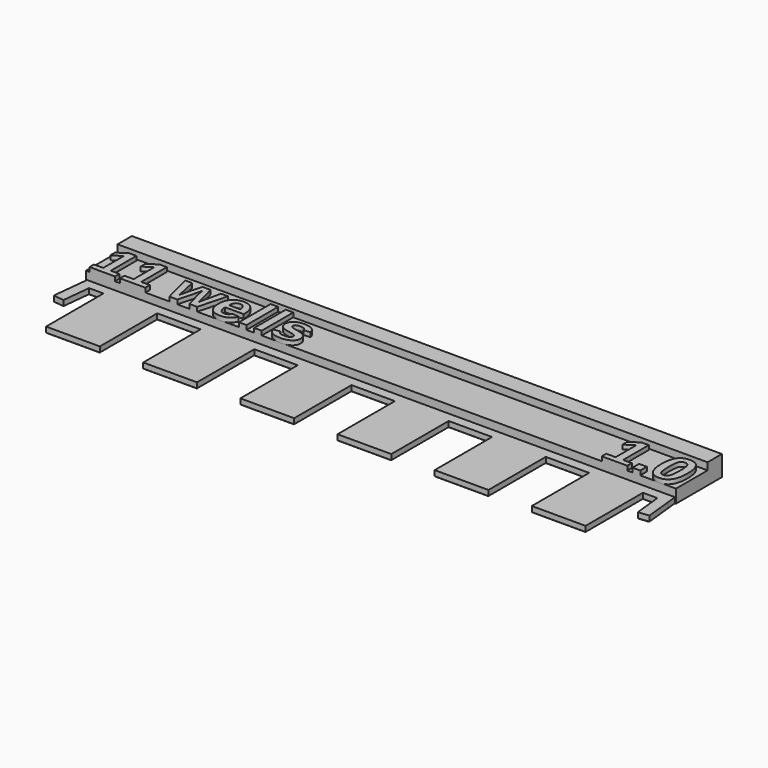
from build123d import *

# Parameters (mm, degrees)
F2_DEPTH      = 0.9
F3_DEPTH      = 2
F1_W          = 82.3
F1_H          = 2.5
F4_DEPTH      = 3
F5_TEXT_SIZE  = 7.6388888889
F6_DEPTH      = 0.6
F7_T1_DEPTH   = 2.532279032
F7_T3_DEPTH   = 10.516139516
F7_T5_DEPTH   = 8.532279032
F7_T7_DEPTH   = 6.05
F7_T9_DEPTH   = 8.532279032
F7_T11_DEPTH  = 6.05
F7_T13_DEPTH  = 8.532279032
F7_T15_DEPTH  = 6.05
F7_T17_DEPTH  = 8.532279032
F7_T19_DEPTH  = 6.05
F7_T21_DEPTH  = 8.532279032
F7_T23_DEPTH  = 6.05
F7_T25_DEPTH  = 8.532279032
F7_T27_DEPTH  = 2.532279032
F7_T29_DEPTH  = 9.032279032
F7_T31_DEPTH  = 83.332279032
F7_T36_DEPTH  = 1.1794249614
F7_T41_DEPTH  = 6.1899906234
F7_T46_DEPTH  = 4.9746099208
F7_T51_DEPTH  = 2.5292526207
F7_T56_DEPTH  = 2.5292526207
F7_T61_DEPTH  = 4.9746099208
F7_T66_DEPTH  = 6.1899906234
F7_T71_DEPTH  = 1.1794249614
F7_T77_DEPTH  = 1.1794249614
F7_T81_DEPTH  = 6.1899906234
F7_T88_DEPTH  = 4.9746099208
F7_T92_DEPTH  = 2.5292526207
F7_T99_DEPTH  = 3.0453921368
F7_T103_DEPTH = 11.032279032
F7_T110_DEPTH = 11.032279032
F7_T114_DEPTH = 6.566139516
F7_T121_DEPTH = 6.566139516
F7_T125_DEPTH = 11.032279032
F7_T132_DEPTH = 11.032279032
F7_T136_DEPTH = 6.566139516
F7_T143_DEPTH = 6.566139516
F7_T147_DEPTH = 11.032279032
F7_T154_DEPTH = 11.032279032
F7_T158_DEPTH = 6.566139516
F7_T165_DEPTH = 6.566139516
F7_T169_DEPTH = 11.032279032
F7_T176_DEPTH = 11.032279032
F7_T180_DEPTH = 6.566139516
F7_T187_DEPTH = 6.566139516
F7_T191_DEPTH = 11.032279032
F7_T198_DEPTH = 11.032279032
F7_T202_DEPTH = 6.566139516
F7_T209_DEPTH = 6.566139516
F7_T213_DEPTH = 11.032279032
F7_T220_DEPTH = 11.032279032
F7_T224_DEPTH = 3.0453921368
F7_T231_DEPTH = 2.5292526207
F7_T235_DEPTH = 4.9746099208
F7_T242_DEPTH = 1.1794249614
F7_T246_DEPTH = 6.1899906234


# Not quite as in the source:
# - a fillet or chamfer that OpenCascade refuses, or shapes differently, is made with other operations: its cross-section is extruded or revolved along the edge and cut away or added
# - Text() gives the source's letters only with a copy of the font that has no kerning and outlines rounded to 1/6400 em; it was checked with that copy


with BuildPart() as f2:
    # F1 (on Top) → F2 (new body)
    with BuildSketch(Plane.XY):
        Polygon((-34.0542682267, 5.1274530911), (-32.041155122, 5.1274530911), (-32.041155122, -4.8725469089), (-24.541155122, -4.8725469089), (-24.541155122, 5.1274530911), (-18.491155122, 5.1274530911), (-18.491155122, -4.8725469089), (-10.991155122, -4.8725469089), (-10.991155122, 5.1274530911), (-4.941155122, 5.1274530911), (-4.941155122, -4.8725469089), (2.558844878, -4.8725469089), (2.558844878, 5.1274530911), (8.608844878, 5.1274530911), (8.608844878, -4.8725469089), (16.108844878, -4.8725469089), (16.108844878, 5.1274530911), (22.158844878, 5.1274530911), (22.158844878, -4.8725469089), (29.658844878, -4.8725469089), (29.658844878, 5.1274530911), (35.708844878, 5.1274530911), (35.708844878, -4.8725469089), (43.208844878, -4.8725469089), (43.208844878, 5.1274530911), (45.2219579827, 5.1274530911), (45.6340437722, 1.2067187034), (47.1258266152, 1.3635113983), (46.733844878, 5.092968506), (46.5866989486, 6.492968506), (-35.4190091927, 6.492968506), (-35.566155122, 5.092968506), (-35.9581368593, 1.3635113983), (-34.4663540162, 1.2067187034), align=None)
    extrude(amount=F2_DEPTH)

    # F1 (on Top) → F3 (join)
    with BuildSketch(Plane.XY):
        Polygon((-35.566155122, 6.492968506), (-35.4190091927, 6.492968506), (46.5866989486, 6.492968506), (46.733844878, 6.492968506), (46.733844878, 11.992968506), (-35.566155122, 11.992968506), align=None)
    extrude(amount=F3_DEPTH)

    # F1 (on Top) → F4 (join)
    with BuildSketch(Plane.XY):
        with Locations((5.583844878, 13.242968506)):
            Rectangle(F1_W, F1_H)
    extrude(amount=F4_DEPTH)

    # F5 (on face) → F6 (join)
    with BuildSketch(Plane.XY.offset(2)):
        with Locations((35.8985584196, 6.492968506)):
            Text('1.0', F5_TEXT_SIZE, font='Arimo', font_style=FontStyle.BOLD, text_align=(TextAlign.LEFT, TextAlign.BOTTOM))
        with Locations((-35.566155122, 6.492968506)):
            Text('11 wells', F5_TEXT_SIZE, font='Arimo', font_style=FontStyle.BOLD, text_align=(TextAlign.LEFT, TextAlign.BOTTOM))
    extrude(amount=F6_DEPTH)

    # F7: chamfer of 0.15 x 0.2 on 36 edges, made by hand

    # F7_s2 → F7_t1 (cut)
    with BuildSketch(Plane(origin=(-36.2203081074, 3.8069077847, 0), x_dir=(0, 0, 1), z_dir=(0.9945218954, -0.1045284633, 0))):
        Polygon((0, 2.2026068477), (0.15, 2.4026068477), (0, 2.4026068477), align=None)
    extrude(amount=F7_T1_DEPTH, mode=Mode.SUBTRACT)

    # F7_s4 → F7_t3 (cut)
    with BuildSketch(Plane.XZ.offset(-5.1274530911)):
        Polygon((-31.841155122, 0), (-32.041155122, 0.15), (-32.041155122, 0), align=None)
        Polygon((-24.741155122, 0), (-24.541155122, 0.15), (-24.541155122, 0), align=None)
        Polygon((-18.291155122, 0), (-18.491155122, 0.15), (-18.491155122, 0), align=None)
        Polygon((-11.191155122, 0), (-10.991155122, 0.15), (-10.991155122, 0), align=None)
        Polygon((-4.741155122, 0), (-4.941155122, 0.15), (-4.941155122, 0), align=None)
        Polygon((2.358844878, 0), (2.558844878, 0.15), (2.558844878, 0), align=None)
        Polygon((8.808844878, 0), (8.608844878, 0.15), (8.608844878, 0), align=None)
        Polygon((15.908844878, 0), (16.108844878, 0.15), (16.108844878, 0), align=None)
        Polygon((22.358844878, 0), (22.158844878, 0.15), (22.158844878, 0), align=None)
        Polygon((29.458844878, 0), (29.658844878, 0.15), (29.658844878, 0), align=None)
        Polygon((35.908844878, 0), (35.708844878, 0.15), (35.708844878, 0), align=None)
        Polygon((43.008844878, 0), (43.208844878, 0.15), (43.208844878, 0), align=None)
    extrude(amount=F7_T3_DEPTH, mode=Mode.SUBTRACT)

    # F7_s6 → F7_t5 (cut)
    with BuildSketch(Plane.YZ.offset(-32.5572946381)):
        Polygon((-4.6725469089, 0), (-4.8725469089, 0.15), (-4.8725469089, 0), align=None)
    extrude(amount=F7_T5_DEPTH, mode=Mode.SUBTRACT)

    # F7_s8 → F7_t7 (cut)
    with BuildSketch(Plane.YZ.offset(-24.541155122)):
        Polygon((5.3274530911, 0), (5.1274530911, 0.15), (5.1274530911, 0), align=None)
    extrude(amount=F7_T7_DEPTH, mode=Mode.SUBTRACT)

    # F7_s10 → F7_t9 (cut)
    with BuildSketch(Plane.YZ.offset(-19.0072946381)):
        Polygon((-4.6725469089, 0), (-4.8725469089, 0.15), (-4.8725469089, 0), align=None)
    extrude(amount=F7_T9_DEPTH, mode=Mode.SUBTRACT)

    # F7_s12 → F7_t11 (cut)
    with BuildSketch(Plane.YZ.offset(-10.991155122)):
        Polygon((5.3274530911, 0), (5.1274530911, 0.15), (5.1274530911, 0), align=None)
    extrude(amount=F7_T11_DEPTH, mode=Mode.SUBTRACT)

    # F7_s14 → F7_t13 (cut)
    with BuildSketch(Plane.YZ.offset(-5.4572946381)):
        Polygon((-4.6725469089, 0), (-4.8725469089, 0.15), (-4.8725469089, 0), align=None)
    extrude(amount=F7_T13_DEPTH, mode=Mode.SUBTRACT)

    # F7_s16 → F7_t15 (cut)
    with BuildSketch(Plane.YZ.offset(2.558844878)):
        Polygon((5.3274530911, 0), (5.1274530911, 0.15), (5.1274530911, 0), align=None)
    extrude(amount=F7_T15_DEPTH, mode=Mode.SUBTRACT)

    # F7_s18 → F7_t17 (cut)
    with BuildSketch(Plane.YZ.offset(8.0927053619)):
        Polygon((-4.6725469089, 0), (-4.8725469089, 0.15), (-4.8725469089, 0), align=None)
    extrude(amount=F7_T17_DEPTH, mode=Mode.SUBTRACT)

    # F7_s20 → F7_t19 (cut)
    with BuildSketch(Plane.YZ.offset(16.108844878)):
        Polygon((5.3274530911, 0), (5.1274530911, 0.15), (5.1274530911, 0), align=None)
    extrude(amount=F7_T19_DEPTH, mode=Mode.SUBTRACT)

    # F7_s22 → F7_t21 (cut)
    with BuildSketch(Plane.YZ.offset(21.6427053619)):
        Polygon((-4.6725469089, 0), (-4.8725469089, 0.15), (-4.8725469089, 0), align=None)
    extrude(amount=F7_T21_DEPTH, mode=Mode.SUBTRACT)

    # F7_s24 → F7_t23 (cut)
    with BuildSketch(Plane.YZ.offset(29.658844878)):
        Polygon((5.3274530911, 0), (5.1274530911, 0.15), (5.1274530911, 0), align=None)
    extrude(amount=F7_T23_DEPTH, mode=Mode.SUBTRACT)

    # F7_s26 → F7_t25 (cut)
    with BuildSketch(Plane.YZ.offset(35.1927053619)):
        Polygon((-4.6725469089, 0), (-4.8725469089, 0.15), (-4.8725469089, 0), align=None)
    extrude(amount=F7_T25_DEPTH, mode=Mode.SUBTRACT)

    # F7_s28 → F7_t27 (cut)
    with BuildSketch(Plane(origin=(44.7475705131, 4.7031591788, 0), x_dir=(0, 0, 1), z_dir=(0.9945218954, 0.1045284633, 0))):
        Polygon((0, 3.3699482961), (0.15, 3.5699482961), (0, 3.5699482961), align=None)
    extrude(amount=F7_T27_DEPTH, mode=Mode.SUBTRACT)

    # F7_s30 → F7_t29 (cut)
    with BuildSketch(Plane.XZ.offset(-15.009108022)):
        Polygon((46.533844878, 0), (46.733844878, 0.15), (46.733844878, 0), align=None)
        Polygon((-35.366155122, 0), (-35.566155122, 0.15), (-35.566155122, 0), align=None)
    extrude(amount=F7_T29_DEPTH, mode=Mode.SUBTRACT)

    # F7_s32 → F7_t31 (cut)
    with BuildSketch(Plane.YZ.offset(-36.0822946381)):
        Polygon((14.292968506, 0), (14.492968506, 0.15), (14.492968506, 0), align=None)
    extrude(amount=F7_T31_DEPTH, mode=Mode.SUBTRACT)


with BuildPart() as f7_tool34:
    # F7_s35 → F7_t36 (new body)
    with BuildSketch(Plane.YZ.offset(-36.0822946381)):
        Polygon((6.492968506, 0.15), (6.692968506, 0), (6.492968506, 0), align=None)
    extrude(amount=F7_T36_DEPTH)

    split(bisect_by=Plane(origin=(-35.7069960577, 3.7529565143, 0), x_dir=(0, 0, 1), z_dir=(-0.9945218954, 0.1045284633, 0)), keep=Keep.TOP)


with BuildPart() as f2_1:
    add(f2.part)

    # F7_t33: cut F7_tool34
    add(f7_tool34.part, mode=Mode.SUBTRACT)


with BuildPart() as f7_tool39:
    # F7_s40 → F7_t41 (new body)
    with BuildSketch(Plane(origin=(0.3419381354, 3.2533240414, 0), x_dir=(0, 0, 1), z_dir=(-0.1045284633, -0.9945218954, 0))):
        Polygon((0, 35.7036801743), (0.15, 35.9036801743), (0, 35.9036801743), align=None)
    extrude(amount=F7_T41_DEPTH)

    split(bisect_by=Plane.XZ.offset(-6.492968506), keep=Keep.TOP)


with BuildPart() as f2_2:
    add(f2_1.part)

    # F7_t38: cut F7_tool39
    add(f7_tool39.part, mode=Mode.SUBTRACT)


with BuildPart() as f7_tool44:
    # F7_s45 → F7_t46 (new body)
    with BuildSketch(Plane(origin=(-0.3050920721, -2.9027571657, 0), x_dir=(0, 0, 1), z_dir=(0.1045284633, 0.9945218954, 0))):
        Polygon((0, -34.6036801743), (0.15, -34.4036801743), (0, -34.4036801743), align=None)
    extrude(amount=F7_T46_DEPTH)

    split(bisect_by=Plane.XZ.offset(-5.1274530911), keep=Keep.TOP)


with BuildPart() as f2_3:
    add(f2_2.part)

    # F7_t43: cut F7_tool44
    add(f7_tool44.part, mode=Mode.SUBTRACT)


with BuildPart() as f7_tool49:
    # F7_s50 → F7_t51 (new body)
    with BuildSketch(Plane.YZ.offset(-34.5704077428)):
        Polygon((5.3274530911, 0), (5.1274530911, 0.15), (5.1274530911, 0), align=None)
    extrude(amount=F7_T51_DEPTH)

    split(bisect_by=Plane(origin=(-34.2152132146, 3.5961638194, 0), x_dir=(0, 0, 1), z_dir=(0.9945218954, -0.1045284633, 0)), keep=Keep.TOP)


with BuildPart() as f2_4:
    add(f2_3.part)

    # F7_t48: cut F7_tool49
    add(f7_tool49.part, mode=Mode.SUBTRACT)


with BuildPart() as f7_tool54:
    # F7_s55 → F7_t56 (new body)
    with BuildSketch(Plane.YZ.offset(43.208844878)):
        Polygon((5.3274530911, 0), (5.1274530911, 0.15), (5.1274530911, 0), align=None)
    extrude(amount=F7_T56_DEPTH)

    split(bisect_by=Plane(origin=(45.2608825628, 4.7571104492, 0), x_dir=(0, 0, 1), z_dir=(-0.9945218954, -0.1045284633, 0)), keep=Keep.TOP)


with BuildPart() as f2_5:
    add(f2_4.part)

    # F7_t53: cut F7_tool54
    add(f7_tool54.part, mode=Mode.SUBTRACT)


with BuildPart() as f7_tool59:
    # F7_s60 → F7_t61 (new body)
    with BuildSketch(Plane(origin=(-0.0928758506, 0.8836546916, 0), x_dir=(0, 0, 1), z_dir=(0.1045284633, -0.9945218954, 0))):
        Polygon((0, -45.7101921573), (0.15, -45.5101921573), (0, -45.5101921573), align=None)
    extrude(amount=F7_T61_DEPTH)

    split(bisect_by=Plane.XZ.offset(-5.1274530911), keep=Keep.TOP)


with BuildPart() as f2_6:
    add(f2_5.part)

    # F7_t58: cut F7_tool59
    add(f7_tool59.part, mode=Mode.SUBTRACT)


with BuildPart() as f7_tool64:
    # F7_s65 → F7_t66 (new body)
    with BuildSketch(Plane(origin=(0.4271124798, -4.0637037955, 0), x_dir=(0, 0, 1), z_dir=(-0.1045284633, 0.9945218954, 0))):
        Polygon((0, 46.8101921573), (0.15, 47.0101921573), (0, 47.0101921573), align=None)
    extrude(amount=F7_T66_DEPTH)

    split(bisect_by=Plane.XZ.offset(-6.492968506), keep=Keep.TOP)


with BuildPart() as f2_7:
    add(f2_6.part)

    # F7_t63: cut F7_tool64
    add(f7_tool64.part, mode=Mode.SUBTRACT)


with BuildPart() as f7_tool69:
    # F7_s70 → F7_t71 (new body)
    with BuildSketch(Plane.YZ.offset(46.0705594326)):
        Polygon((6.492968506, 0.15), (6.692968506, 0), (6.492968506, 0), align=None)
    extrude(amount=F7_T71_DEPTH)

    split(bisect_by=Plane(origin=(46.7526654059, 4.9139031441, 0), x_dir=(0, 0, 1), z_dir=(0.9945218954, 0.1045284633, 0)), keep=Keep.TOP)


with BuildPart() as f2_8:
    add(f2_7.part)

    # F7_t68: cut F7_tool69
    add(f7_tool69.part, mode=Mode.SUBTRACT)


with BuildPart() as f7_tool75:
    # F7_s76 → F7_t77 (new body)
    with BuildSketch(Plane.YZ.offset(-36.0822946381)):
        Polygon((6.492968506, 0.15), (6.692968506, 0), (6.492968506, 0), align=None)
    extrude(amount=F7_T77_DEPTH)

    split(bisect_by=Plane(origin=(-35.7069960577, 3.7529565143, 0), x_dir=(0, 0, 1), z_dir=(0.9945218954, -0.1045284633, 0)), keep=Keep.TOP)


with BuildPart() as f7_tool79:
    # F7_s80 → F7_t81 (new body)
    with BuildSketch(Plane(origin=(0.3419381354, 3.2533240414, 0), x_dir=(0, 0, 1), z_dir=(-0.1045284633, -0.9945218954, 0))):
        Polygon((0, 35.7036801743), (0.15, 35.9036801743), (0, 35.9036801743), align=None)
    extrude(amount=F7_T81_DEPTH)

    split(bisect_by=Plane.XZ.offset(-6.492968506), keep=Keep.BOTTOM)


with BuildPart() as f7_tool75_1:
    add(f7_tool75.part)

    # F7_t83: intersect F7_tool79
    add(f7_tool79.part, mode=Mode.INTERSECT)


with BuildPart() as f2_9:
    add(f2_8.part)

    # F7_t73: cut F7_tool75
    add(f7_tool75_1.part, mode=Mode.SUBTRACT)


with BuildPart() as f7_tool86:
    # F7_s87 → F7_t88 (new body)
    with BuildSketch(Plane(origin=(-0.3050920721, -2.9027571657, 0), x_dir=(0, 0, 1), z_dir=(0.1045284633, 0.9945218954, 0))):
        Polygon((0, -34.6036801743), (0.15, -34.4036801743), (0, -34.4036801743), align=None)
    extrude(amount=F7_T88_DEPTH)

    split(bisect_by=Plane.XZ.offset(-5.1274530911), keep=Keep.BOTTOM)


with BuildPart() as f7_tool90:
    # F7_s91 → F7_t92 (new body)
    with BuildSketch(Plane.YZ.offset(-34.5704077428)):
        Polygon((5.3274530911, 0), (5.1274530911, 0.15), (5.1274530911, 0), align=None)
    extrude(amount=F7_T92_DEPTH)

    split(bisect_by=Plane(origin=(-34.2152132146, 3.5961638194, 0), x_dir=(0, 0, 1), z_dir=(-0.9945218954, 0.1045284633, 0)), keep=Keep.TOP)


with BuildPart() as f7_tool86_1:
    add(f7_tool86.part)

    # F7_t94: intersect F7_tool90
    add(f7_tool90.part, mode=Mode.INTERSECT)


with BuildPart() as f2_10:
    add(f2_9.part)

    # F7_t84: cut F7_tool86
    add(f7_tool86_1.part, mode=Mode.SUBTRACT)


with BuildPart() as f7_tool97:
    # F7_s98 → F7_t99 (new body)
    with BuildSketch(Plane.YZ.offset(-34.5704077428)):
        Polygon((5.3274530911, 0), (5.1274530911, 0.15), (5.1274530911, 0), align=None)
    extrude(amount=F7_T99_DEPTH)

    split(bisect_by=Plane.YZ.offset(-32.041155122), keep=Keep.TOP)


with BuildPart() as f7_tool101:
    # F7_s102 → F7_t103 (new body)
    with BuildSketch(Plane.XZ.offset(-5.6435926071)):
        Polygon((-31.841155122, 0), (-32.041155122, 0.15), (-32.041155122, 0), align=None)
    extrude(amount=F7_T103_DEPTH)

    split(bisect_by=Plane.XZ.offset(-5.1274530911), keep=Keep.BOTTOM)


with BuildPart() as f7_tool97_1:
    add(f7_tool97.part)

    # F7_t105: intersect F7_tool101
    add(f7_tool101.part, mode=Mode.INTERSECT)


with BuildPart() as f2_11:
    add(f2_10.part)

    # F7_t95: cut F7_tool97
    add(f7_tool97_1.part, mode=Mode.SUBTRACT)


with BuildPart() as f7_tool108:
    # F7_s109 → F7_t110 (new body)
    with BuildSketch(Plane.XZ.offset(5.3886864249)):
        Polygon((-24.741155122, 0), (-24.541155122, 0.15), (-24.541155122, 0), align=None)
    extrude(amount=-F7_T110_DEPTH)

    split(bisect_by=Plane.XZ.offset(-5.1274530911), keep=Keep.BOTTOM)


with BuildPart() as f7_tool112:
    # F7_s113 → F7_t114 (new body)
    with BuildSketch(Plane.YZ.offset(-25.0572946381)):
        Polygon((5.3274530911, 0), (5.1274530911, 0.15), (5.1274530911, 0), align=None)
    extrude(amount=F7_T114_DEPTH)

    split(bisect_by=Plane.YZ.offset(-24.541155122), keep=Keep.BOTTOM)


with BuildPart() as f7_tool108_1:
    add(f7_tool108.part)

    # F7_t116: intersect F7_tool112
    add(f7_tool112.part, mode=Mode.INTERSECT)


with BuildPart() as f2_12:
    add(f2_11.part)

    # F7_t106: cut F7_tool108
    add(f7_tool108_1.part, mode=Mode.SUBTRACT)


with BuildPart() as f7_tool119:
    # F7_s120 → F7_t121 (new body)
    with BuildSketch(Plane.YZ.offset(-24.541155122)):
        Polygon((5.3274530911, 0), (5.1274530911, 0.15), (5.1274530911, 0), align=None)
    extrude(amount=F7_T121_DEPTH)

    split(bisect_by=Plane.YZ.offset(-18.491155122), keep=Keep.TOP)


with BuildPart() as f7_tool123:
    # F7_s124 → F7_t125 (new body)
    with BuildSketch(Plane.XZ.offset(-5.6435926071)):
        Polygon((-18.291155122, 0), (-18.491155122, 0.15), (-18.491155122, 0), align=None)
    extrude(amount=F7_T125_DEPTH)

    split(bisect_by=Plane.XZ.offset(-5.1274530911), keep=Keep.BOTTOM)


with BuildPart() as f7_tool119_1:
    add(f7_tool119.part)

    # F7_t127: intersect F7_tool123
    add(f7_tool123.part, mode=Mode.INTERSECT)


with BuildPart() as f2_13:
    add(f2_12.part)

    # F7_t117: cut F7_tool119
    add(f7_tool119_1.part, mode=Mode.SUBTRACT)


with BuildPart() as f7_tool130:
    # F7_s131 → F7_t132 (new body)
    with BuildSketch(Plane.XZ.offset(5.3886864249)):
        Polygon((-11.191155122, 0), (-10.991155122, 0.15), (-10.991155122, 0), align=None)
    extrude(amount=-F7_T132_DEPTH)

    split(bisect_by=Plane.XZ.offset(-5.1274530911), keep=Keep.BOTTOM)


with BuildPart() as f7_tool134:
    # F7_s135 → F7_t136 (new body)
    with BuildSketch(Plane.YZ.offset(-11.5072946381)):
        Polygon((5.3274530911, 0), (5.1274530911, 0.15), (5.1274530911, 0), align=None)
    extrude(amount=F7_T136_DEPTH)

    split(bisect_by=Plane.YZ.offset(-10.991155122), keep=Keep.BOTTOM)


with BuildPart() as f7_tool130_1:
    add(f7_tool130.part)

    # F7_t138: intersect F7_tool134
    add(f7_tool134.part, mode=Mode.INTERSECT)


with BuildPart() as f2_14:
    add(f2_13.part)

    # F7_t128: cut F7_tool130
    add(f7_tool130_1.part, mode=Mode.SUBTRACT)


with BuildPart() as f7_tool141:
    # F7_s142 → F7_t143 (new body)
    with BuildSketch(Plane.YZ.offset(-10.991155122)):
        Polygon((5.3274530911, 0), (5.1274530911, 0.15), (5.1274530911, 0), align=None)
    extrude(amount=F7_T143_DEPTH)

    split(bisect_by=Plane.YZ.offset(-4.941155122), keep=Keep.TOP)


with BuildPart() as f7_tool145:
    # F7_s146 → F7_t147 (new body)
    with BuildSketch(Plane.XZ.offset(-5.6435926071)):
        Polygon((-4.741155122, 0), (-4.941155122, 0.15), (-4.941155122, 0), align=None)
    extrude(amount=F7_T147_DEPTH)

    split(bisect_by=Plane.XZ.offset(-5.1274530911), keep=Keep.BOTTOM)


with BuildPart() as f7_tool141_1:
    add(f7_tool141.part)

    # F7_t149: intersect F7_tool145
    add(f7_tool145.part, mode=Mode.INTERSECT)


with BuildPart() as f2_15:
    add(f2_14.part)

    # F7_t139: cut F7_tool141
    add(f7_tool141_1.part, mode=Mode.SUBTRACT)


with BuildPart() as f7_tool152:
    # F7_s153 → F7_t154 (new body)
    with BuildSketch(Plane.XZ.offset(5.3886864249)):
        Polygon((2.358844878, 0), (2.558844878, 0.15), (2.558844878, 0), align=None)
    extrude(amount=-F7_T154_DEPTH)

    split(bisect_by=Plane.XZ.offset(-5.1274530911), keep=Keep.BOTTOM)


with BuildPart() as f7_tool156:
    # F7_s157 → F7_t158 (new body)
    with BuildSketch(Plane.YZ.offset(2.0427053619)):
        Polygon((5.3274530911, 0), (5.1274530911, 0.15), (5.1274530911, 0), align=None)
    extrude(amount=F7_T158_DEPTH)

    split(bisect_by=Plane.YZ.offset(2.558844878), keep=Keep.BOTTOM)


with BuildPart() as f7_tool152_1:
    add(f7_tool152.part)

    # F7_t160: intersect F7_tool156
    add(f7_tool156.part, mode=Mode.INTERSECT)


with BuildPart() as f2_16:
    add(f2_15.part)

    # F7_t150: cut F7_tool152
    add(f7_tool152_1.part, mode=Mode.SUBTRACT)


with BuildPart() as f7_tool163:
    # F7_s164 → F7_t165 (new body)
    with BuildSketch(Plane.YZ.offset(2.558844878)):
        Polygon((5.3274530911, 0), (5.1274530911, 0.15), (5.1274530911, 0), align=None)
    extrude(amount=F7_T165_DEPTH)

    split(bisect_by=Plane.YZ.offset(8.608844878), keep=Keep.TOP)


with BuildPart() as f7_tool167:
    # F7_s168 → F7_t169 (new body)
    with BuildSketch(Plane.XZ.offset(-5.6435926071)):
        Polygon((8.808844878, 0), (8.608844878, 0.15), (8.608844878, 0), align=None)
    extrude(amount=F7_T169_DEPTH)

    split(bisect_by=Plane.XZ.offset(-5.1274530911), keep=Keep.BOTTOM)


with BuildPart() as f7_tool163_1:
    add(f7_tool163.part)

    # F7_t171: intersect F7_tool167
    add(f7_tool167.part, mode=Mode.INTERSECT)


with BuildPart() as f2_17:
    add(f2_16.part)

    # F7_t161: cut F7_tool163
    add(f7_tool163_1.part, mode=Mode.SUBTRACT)


with BuildPart() as f7_tool174:
    # F7_s175 → F7_t176 (new body)
    with BuildSketch(Plane.XZ.offset(5.3886864249)):
        Polygon((15.908844878, 0), (16.108844878, 0.15), (16.108844878, 0), align=None)
    extrude(amount=-F7_T176_DEPTH)

    split(bisect_by=Plane.XZ.offset(-5.1274530911), keep=Keep.BOTTOM)


with BuildPart() as f7_tool178:
    # F7_s179 → F7_t180 (new body)
    with BuildSketch(Plane.YZ.offset(15.5927053619)):
        Polygon((5.3274530911, 0), (5.1274530911, 0.15), (5.1274530911, 0), align=None)
    extrude(amount=F7_T180_DEPTH)

    split(bisect_by=Plane.YZ.offset(16.108844878), keep=Keep.BOTTOM)


with BuildPart() as f7_tool174_1:
    add(f7_tool174.part)

    # F7_t182: intersect F7_tool178
    add(f7_tool178.part, mode=Mode.INTERSECT)


with BuildPart() as f2_18:
    add(f2_17.part)

    # F7_t172: cut F7_tool174
    add(f7_tool174_1.part, mode=Mode.SUBTRACT)


with BuildPart() as f7_tool185:
    # F7_s186 → F7_t187 (new body)
    with BuildSketch(Plane.YZ.offset(16.108844878)):
        Polygon((5.3274530911, 0), (5.1274530911, 0.15), (5.1274530911, 0), align=None)
    extrude(amount=F7_T187_DEPTH)

    split(bisect_by=Plane.YZ.offset(22.158844878), keep=Keep.TOP)


with BuildPart() as f7_tool189:
    # F7_s190 → F7_t191 (new body)
    with BuildSketch(Plane.XZ.offset(-5.6435926071)):
        Polygon((22.358844878, 0), (22.158844878, 0.15), (22.158844878, 0), align=None)
    extrude(amount=F7_T191_DEPTH)

    split(bisect_by=Plane.XZ.offset(-5.1274530911), keep=Keep.BOTTOM)


with BuildPart() as f7_tool185_1:
    add(f7_tool185.part)

    # F7_t193: intersect F7_tool189
    add(f7_tool189.part, mode=Mode.INTERSECT)


with BuildPart() as f2_19:
    add(f2_18.part)

    # F7_t183: cut F7_tool185
    add(f7_tool185_1.part, mode=Mode.SUBTRACT)


with BuildPart() as f7_tool196:
    # F7_s197 → F7_t198 (new body)
    with BuildSketch(Plane.XZ.offset(5.3886864249)):
        Polygon((29.458844878, 0), (29.658844878, 0.15), (29.658844878, 0), align=None)
    extrude(amount=-F7_T198_DEPTH)

    split(bisect_by=Plane.XZ.offset(-5.1274530911), keep=Keep.BOTTOM)


with BuildPart() as f7_tool200:
    # F7_s201 → F7_t202 (new body)
    with BuildSketch(Plane.YZ.offset(29.1427053619)):
        Polygon((5.3274530911, 0), (5.1274530911, 0.15), (5.1274530911, 0), align=None)
    extrude(amount=F7_T202_DEPTH)

    split(bisect_by=Plane.YZ.offset(29.658844878), keep=Keep.BOTTOM)


with BuildPart() as f7_tool196_1:
    add(f7_tool196.part)

    # F7_t204: intersect F7_tool200
    add(f7_tool200.part, mode=Mode.INTERSECT)


with BuildPart() as f2_20:
    add(f2_19.part)

    # F7_t194: cut F7_tool196
    add(f7_tool196_1.part, mode=Mode.SUBTRACT)


with BuildPart() as f7_tool207:
    # F7_s208 → F7_t209 (new body)
    with BuildSketch(Plane.YZ.offset(29.658844878)):
        Polygon((5.3274530911, 0), (5.1274530911, 0.15), (5.1274530911, 0), align=None)
    extrude(amount=F7_T209_DEPTH)

    split(bisect_by=Plane.YZ.offset(35.708844878), keep=Keep.TOP)


with BuildPart() as f7_tool211:
    # F7_s212 → F7_t213 (new body)
    with BuildSketch(Plane.XZ.offset(-5.6435926071)):
        Polygon((35.908844878, 0), (35.708844878, 0.15), (35.708844878, 0), align=None)
    extrude(amount=F7_T213_DEPTH)

    split(bisect_by=Plane.XZ.offset(-5.1274530911), keep=Keep.BOTTOM)


with BuildPart() as f7_tool207_1:
    add(f7_tool207.part)

    # F7_t215: intersect F7_tool211
    add(f7_tool211.part, mode=Mode.INTERSECT)


with BuildPart() as f2_21:
    add(f2_20.part)

    # F7_t205: cut F7_tool207
    add(f7_tool207_1.part, mode=Mode.SUBTRACT)


with BuildPart() as f7_tool218:
    # F7_s219 → F7_t220 (new body)
    with BuildSketch(Plane.XZ.offset(5.3886864249)):
        Polygon((43.008844878, 0), (43.208844878, 0.15), (43.208844878, 0), align=None)
    extrude(amount=-F7_T220_DEPTH)

    split(bisect_by=Plane.XZ.offset(-5.1274530911), keep=Keep.BOTTOM)


with BuildPart() as f7_tool222:
    # F7_s223 → F7_t224 (new body)
    with BuildSketch(Plane.YZ.offset(42.6927053619)):
        Polygon((5.3274530911, 0), (5.1274530911, 0.15), (5.1274530911, 0), align=None)
    extrude(amount=F7_T224_DEPTH)

    split(bisect_by=Plane.YZ.offset(43.208844878), keep=Keep.BOTTOM)


with BuildPart() as f7_tool218_1:
    add(f7_tool218.part)

    # F7_t226: intersect F7_tool222
    add(f7_tool222.part, mode=Mode.INTERSECT)


with BuildPart() as f2_22:
    add(f2_21.part)

    # F7_t216: cut F7_tool218
    add(f7_tool218_1.part, mode=Mode.SUBTRACT)


with BuildPart() as f7_tool229:
    # F7_s230 → F7_t231 (new body)
    with BuildSketch(Plane.YZ.offset(43.208844878)):
        Polygon((5.3274530911, 0), (5.1274530911, 0.15), (5.1274530911, 0), align=None)
    extrude(amount=F7_T231_DEPTH)

    split(bisect_by=Plane(origin=(45.2608825628, 4.7571104492, 0), x_dir=(0, 0, 1), z_dir=(0.9945218954, 0.1045284633, 0)), keep=Keep.TOP)


with BuildPart() as f7_tool233:
    # F7_s234 → F7_t235 (new body)
    with BuildSketch(Plane(origin=(-0.0928758506, 0.8836546916, 0), x_dir=(0, 0, 1), z_dir=(0.1045284633, -0.9945218954, 0))):
        Polygon((0, -45.7101921573), (0.15, -45.5101921573), (0, -45.5101921573), align=None)
    extrude(amount=F7_T235_DEPTH)

    split(bisect_by=Plane.XZ.offset(-5.1274530911), keep=Keep.BOTTOM)


with BuildPart() as f7_tool229_1:
    add(f7_tool229.part)

    # F7_t237: intersect F7_tool233
    add(f7_tool233.part, mode=Mode.INTERSECT)


with BuildPart() as f2_23:
    add(f2_22.part)

    # F7_t227: cut F7_tool229
    add(f7_tool229_1.part, mode=Mode.SUBTRACT)


with BuildPart() as f7_tool240:
    # F7_s241 → F7_t242 (new body)
    with BuildSketch(Plane.YZ.offset(46.0705594326)):
        Polygon((6.492968506, 0.15), (6.692968506, 0), (6.492968506, 0), align=None)
    extrude(amount=F7_T242_DEPTH)

    split(bisect_by=Plane(origin=(46.7526654059, 4.9139031441, 0), x_dir=(0, 0, 1), z_dir=(-0.9945218954, -0.1045284633, 0)), keep=Keep.TOP)


with BuildPart() as f7_tool244:
    # F7_s245 → F7_t246 (new body)
    with BuildSketch(Plane(origin=(0.4271124798, -4.0637037955, 0), x_dir=(0, 0, 1), z_dir=(-0.1045284633, 0.9945218954, 0))):
        Polygon((0, 46.8101921573), (0.15, 47.0101921573), (0, 47.0101921573), align=None)
    extrude(amount=F7_T246_DEPTH)

    split(bisect_by=Plane.XZ.offset(-6.492968506), keep=Keep.BOTTOM)


with BuildPart() as f7_tool240_1:
    add(f7_tool240.part)

    # F7_t248: intersect F7_tool244
    add(f7_tool244.part, mode=Mode.INTERSECT)


with BuildPart() as f2_24:
    add(f2_23.part)

    # F7_t238: cut F7_tool240
    add(f7_tool240_1.part, mode=Mode.SUBTRACT)


solid = f2_24.part
